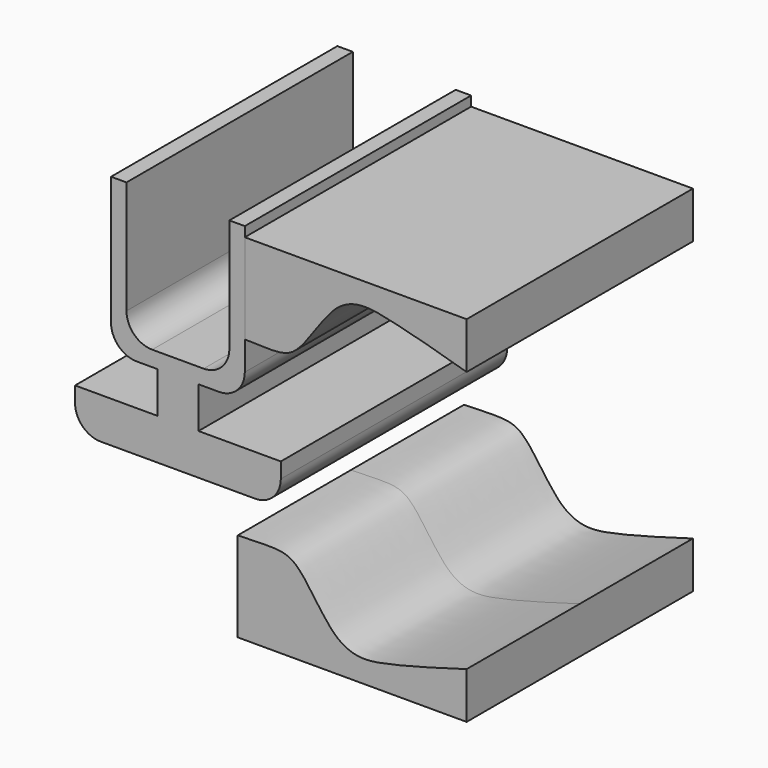
from build123d import *

# Parameters (mm, degrees)
F0_W     = 8
F0_H     = 8
F1_DEPTH = 27.5
F2_R     = 5
F4_DEPTH = 27.5


# Not quite as in the source:
# - ends of sketch curves that miss each other by under 0.0002 mm in the source are joined
# - the dataset's text gives a spline's control points without its knots; the knots are read off the source's solid


with BuildPart() as f1:
    # F0 (on Front) → F1 (new body, symmetric)
    with BuildSketch(Plane.XZ):
        Polygon((4, -1.6261266097), (-4, -1.6261266097), (-20, -1.6261266097), (-20, -9.6261266097), (20, -9.6261266097), (20, -1.6261266097), align=None)
        with Locations((0, 2.3738733903)):
            Rectangle(F0_W, F0_H)
        Polygon((10, 9.3738733903), (-10, 9.3738733903), (-10, 6.3738733903), (-4, 6.3738733903), (4, 6.3738733903), (10, 6.3738733903), align=None)
        Polygon((10, 36.3738733903), (10, 9.3738733903), (10, 6.3738733903), (13, 6.3738733903), (13, 36.3738733903), align=None)
        Polygon((-10, 6.3738733903), (-10, 9.3738733903), (-10, 36.3738733903), (-13, 36.3738733903), (-13, 6.3738733903), align=None)
    extrude(amount=F1_DEPTH, both=True)

    # F2
    f2_edges = [f1.edges().sort_by_distance(p)[0] for p in [
        (-10, 0, 9.373873),
        (10, 0, 9.373873),
        (-13, 0, 6.373873),
        (13, 0, 6.373873),
        (-20, 0, -9.626127),
        (20, 0, -9.626127),
    ]]
    fillet(f2_edges, radius=F2_R)


with BuildPart() as f4:
    # F3 (on face) → F4 (new body, symmetric)
    with BuildSketch(Plane.XZ):
        with BuildLine():
            add(Edge.make_bspline(
                [(13, 16.982425441), (13.3221049388, 16.975283085), (14.2468621208, 16.9493397661), (15.6703167752, 16.8959724351), (17.1878938179, 16.8532591399), (18.5197595049, 16.8637345138), (19.661148945, 16.9499224444), (20.6173837451, 17.1219904621), (21.4182121622, 17.3811060261), (22.0173616007, 17.6864167687), (22.4884805808, 18.0076637751), (22.8744037832, 18.319289904), (23.286877997, 18.7005844423), (23.8614996186, 19.2931691448), (24.6116337326, 20.1740111556), (25.5346734896, 21.391087418), (26.469962642, 22.7050877575), (27.4176091079, 24.0576889473), (28.3873048369, 25.3967470048), (29.4036658306, 26.678135584), (30.327491453, 27.6686536176), (31.1729825946, 28.3976028868), (31.8470413129, 28.8805098687), (32.5627740763, 29.2941269064), (33.5631755653, 29.7402923218), (34.8658914075, 30.0822908079), (36.3929895279, 30.1828251322), (37.8542569952, 30.0777961017), (39.0598071597, 29.8861534433), (40.0466828495, 29.6947045241), (41.0693354085, 29.4809303507), (42.4270502919, 29.1726033038), (44.1407063903, 28.7537628592), (45.8989174866, 28.3017669607), (47.6573517935, 27.8330158596), (49.3709017945, 27.3639959763), (50.9934781418, 26.9113753741), (52.2307294973, 26.5619135441), (53.1278397778, 26.307471025), (53.7476502781, 26.1315623549), (54.3100968987, 25.9721366565), (54.8007807594, 25.8341146441), (55.2551563813, 25.7060591758), (55.6898163291, 25.5771097939), (55.9825851302, 25.4806270935), (56.1303042563, 25.427580175)],
                knots=[0.2575795272, 0.2575795272, 0.2575795272, 0.2575795272, 0.265625, 0.28125, 0.296875, 0.3125, 0.328125, 0.34375, 0.359375, 0.375, 0.3828125, 0.390625, 0.3984375, 0.40625, 0.421875, 0.4375, 0.453125, 0.46875, 0.484375, 0.5, 0.515625, 0.5234375, 0.53125, 0.5390625, 0.546875, 0.5625, 0.578125, 0.59375, 0.609375, 0.6171875, 0.625, 0.640625, 0.65625, 0.671875, 0.6875, 0.703125, 0.71875, 0.734375, 0.7421875, 0.75, 0.7578125, 0.765625, 0.7734375, 0.78125, 0.7887563115, 0.7887563115, 0.7887563115, 0.7887563115], degree=3))
            Line((56.1303043281, 25.427580175), (56.1303043281, 34.4637259841))
            Line((56.1303043281, 34.4637259841), (13, 34.4637259841))
            Line((13, 34.4637259841), (13, 16.982425441))
        make_face()
    extrude(amount=F4_DEPTH, both=True)


with BuildPart() as f4b:
    # F3 (on face) → F4, piece 2 (new body, symmetric)
    with BuildSketch(Plane.XZ):
        with BuildLine():
            Line((56.1303043281, -34.4637259841), (56.1303043281, -25.427580175))
            add(Edge.make_bspline(
                [(11.630304461, -16.9999345971), (11.7777588517, -16.9995671606), (12.5846230757, -16.9947640308), (13.9722983487, -16.9596335508), (15.6703167752, -16.8959724351), (17.1878938179, -16.8532591399), (18.5197595049, -16.8637345138), (19.661148945, -16.9499224444), (20.6173837451, -17.1219904621), (21.4182121622, -17.3811060261), (22.0173616007, -17.6864167687), (22.4884805808, -18.0076637751), (22.8744037832, -18.319289904), (23.286877997, -18.7005844423), (23.8614996186, -19.2931691448), (24.6116337326, -20.1740111556), (25.5346734896, -21.391087418), (26.469962642, -22.7050877575), (27.4176091079, -24.0576889473), (28.3873048369, -25.3967470048), (29.4036658306, -26.678135584), (30.327491453, -27.6686536176), (31.1729825946, -28.3976028868), (31.8470413129, -28.8805098687), (32.5627740763, -29.2941269064), (33.5631755653, -29.7402923218), (34.8658914075, -30.0822908079), (36.3929895279, -30.1828251322), (37.8542569952, -30.0777961017), (39.0598071597, -29.8861534433), (40.0466828495, -29.6947045241), (41.0693354085, -29.4809303507), (42.4270502919, -29.1726033038), (44.1407063903, -28.7537628592), (45.8989174866, -28.3017669607), (47.6573517935, -27.8330158596), (49.3709017945, -27.3639959763), (50.9934781418, -26.9113753741), (52.2307294973, -26.5619135441), (53.1278397778, -26.307471025), (53.7476502781, -26.1315623549), (54.3100968987, -25.9721366565), (54.8007807594, -25.8341146441), (55.2551563813, -25.7060591758), (55.6898163291, -25.5771097939), (55.9825851302, -25.4806270935), (56.1303043281, -25.427580175)],
                knots=[0.2465394652, 0.2465394652, 0.2465394652, 0.2465394652, 0.25, 0.265625, 0.28125, 0.296875, 0.3125, 0.328125, 0.34375, 0.359375, 0.375, 0.3828125, 0.390625, 0.3984375, 0.40625, 0.421875, 0.4375, 0.453125, 0.46875, 0.484375, 0.5, 0.515625, 0.5234375, 0.53125, 0.5390625, 0.546875, 0.5625, 0.578125, 0.59375, 0.609375, 0.6171875, 0.625, 0.640625, 0.65625, 0.671875, 0.6875, 0.703125, 0.71875, 0.734375, 0.7421875, 0.75, 0.7578125, 0.765625, 0.7734375, 0.78125, 0.7887563115, 0.7887563115, 0.7887563115, 0.7887563115], degree=3))
            Line((11.630304461, -16.9999345971), (11.6303046489, -34.4637259841))
            Line((11.6303046489, -34.4637259841), (56.1303043281, -34.4637259841))
        make_face()
    extrude(amount=F4_DEPTH, both=True)


solid = Compound([f1.part, f4.part, f4b.part])
